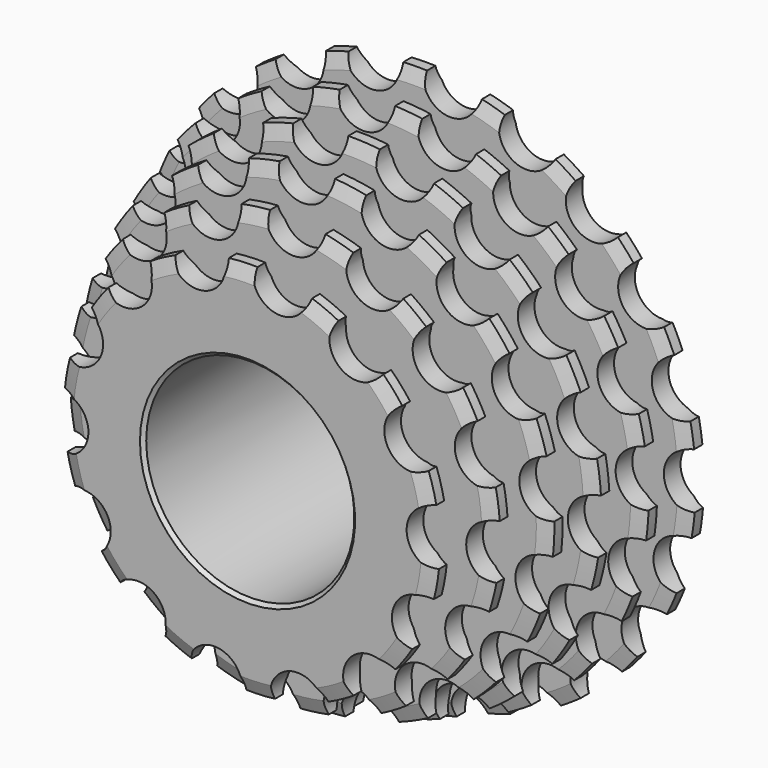
from build123d import *

# Parameters (mm, degrees)
F0_R        = 15
F1_DEPTH    = 3
F2_SIZE2    = 0.75
F2_SIZE     = 2
F2_2_SIZE2  = 0.75
F2_2_SIZE   = 2
F4_SIZE     = 0.5
F5_R        = 17.5
F6_DEPTH    = 3
F7_R        = 38.0209406439
F8_DEPTH    = 3
F9_SIZE2    = 0.75
F9_SIZE     = 2
F9_2_SIZE2  = 0.75
F9_2_SIZE   = 2
F10_R       = 4
F11_DEPTH   = 3
F12_R       = 17.5
F13_DEPTH   = 3
F14_R       = 36.0043728374
F15_DEPTH   = 3
F16_SIZE2   = 2
F16_SIZE    = 0.75
F17_R       = 4
F18_DEPTH   = 3
F19_R       = 17.5
F20_DEPTH   = 3
F21_R       = 34.0193951986
F22_DEPTH   = 3
F23_SIZE2   = 2
F23_SIZE    = 0.75
F24_R       = 4
F25_DEPTH   = 3
F26_R       = 17.5
F27_DEPTH   = 3
F28_R       = 30.9833920726
F29_DEPTH   = 3
F30_SIZE2   = 0.8
F30_SIZE    = 2
F30_2_SIZE2 = 0.8
F30_2_SIZE  = 2
F31_R       = 4
F32_DEPTH   = 3
F33_R       = 17.5
F34_DEPTH   = 3
F35_R       = 27.0849501577
F36_DEPTH   = 3
F37_SIZE2   = 0.8
F37_SIZE    = 2
F37_2_SIZE2 = 0.8
F37_2_SIZE  = 2
F38_R       = 4
F39_DEPTH   = 3
F40_R       = 15
F41_DEPTH   = 30.0010001
F42_SIZE    = 0.5


# Not quite as in the source:
# - two fillets or chamfers of one size are made in one step


with BuildPart() as f1:
    # F0 (on Front) → F1 (new body)
    with BuildSketch(Plane.XZ):
        with BuildLine():
            ThreePointArc((39.8415623905, -3.556670674), (35.9978191055, 0.3962570459), (39.7536154095, 4.4328390311))
            ThreePointArc((39.7536154095, 4.4328390311), (39.5277999491, 6.1280528053), (39.2297290943, 7.8120647197))
            ThreePointArc((39.2297290943, 7.8120647197), (34.4280159865, 10.5219634686), (36.8944395869, 15.4531656165))
            ThreePointArc((36.8944395869, 15.4531656165), (36.2001743283, 17.0160917546), (35.4397364551, 18.5479130899))
            ThreePointArc((35.4397364551, 18.5479130899), (30.0690597635, 19.7952429876), (31.0462956886, 25.2215686272))
            ThreePointArc((31.0462956886, 25.2215686272), (29.9398258742, 26.5255881485), (28.7786271366, 27.7811198502))
            ThreePointArc((28.7786271366, 27.7811198502), (23.2740871461, 27.4648296466), (22.6829655531, 32.9466701461))
            ThreePointArc((22.6829655531, 32.9466701461), (21.2539307867, 33.8861391444), (19.7860446005, 34.763665501))
            ThreePointArc((19.7860446005, 34.763665501), (14.5935864044, 32.9093791473), (12.4819964492, 38.0026283912))
            ThreePointArc((12.4819964492, 38.0026283912), (10.8461686289, 38.5014366755), (9.190514403, 38.9298657204))
            ThreePointArc((9.190514403, 38.9298657204), (4.7308000836, 35.687806469), (1.2698102264, 39.9798396944))
            ThreePointArc((1.2698102264, 39.9798396944), (-0.4402856066, 39.9975767839), (-2.1495766133, 39.9421997439))
            ThreePointArc((-2.1495766133, 39.9421997439), (-2.1334373815, 39.7352791434), (-2.1280528053, 39.5277999491))
            ThreePointArc((-2.1280528053, 39.5277999491), (-5.7211023511, 35.548554879), (-10.0452484692, 38.7181221548))
            ThreePointArc((-10.0452484692, 38.7181221548), (-11.6910705207, 38.2533510961), (-13.3155217164, 37.7186542896))
            ThreePointArc((-13.3155217164, 37.7186542896), (-13.091663124, 36.9740347316), (-13.0160917546, 36.2001743283))
            ThreePointArc((-13.0160917546, 36.2001743283), (-16.0469778506, 32.3193473235), (-20.5465008752, 34.3196926237))
            ThreePointArc((-20.5465008752, 34.3196926237), (-21.9947144307, 33.4100664039), (-23.4027224406, 32.4393677862))
            ThreePointArc((-23.4027224406, 32.4393677862), (-22.751236361, 31.2643139202), (-22.5255881485, 29.9398258742))
            ThreePointArc((-22.5255881485, 29.9398258742), (-25.0140391592, 26.2364193811), (-29.383197975, 27.1408857034))
            ThreePointArc((-29.383197975, 27.1408857034), (-30.5164773851, 25.860096829), (-31.5939737739, 24.5320366291))
            ThreePointArc((-31.5939737739, 24.5320366291), (-30.338699118, 23.1020837184), (-29.8861391444, 21.2539307867))
            ThreePointArc((-29.8861391444, 21.2539307867), (-31.8629258482, 17.8033354818), (-35.8394431235, 17.7632856364))
            ThreePointArc((-35.8394431235, 17.7632856364), (-36.5659768303, 16.2150960049), (-37.2256692487, 14.637265762))
            ThreePointArc((-37.2256692487, 14.637265762), (-35.2531240591, 13.1803633822), (-34.5014366755, 10.8461686289))
            ThreePointArc((-34.5014366755, 10.8461686289), (-36.0077458606, 7.7186286819), (-39.3921897355, 6.9466098095))
            ThreePointArc((-39.3921897355, 6.9466098095), (-39.6531182989, 5.2564445374), (-39.8415623905, 3.556670674))
            ThreePointArc((-39.8415623905, 3.556670674), (-37.1145178551, 2.3324334944), (-35.9975767839, -0.4402856066))
            ThreePointArc((-35.9975767839, -0.4402856066), (-37.0841728042, -3.1811025014), (-39.7536154095, -4.4328390311))
            ThreePointArc((-39.7536154095, -4.4328390311), (-39.5277999491, -6.1280528053), (-39.2297290943, -7.8120647197))
            ThreePointArc((-39.2297290943, -7.8120647197), (-35.7942366206, -8.536271637), (-34.2533510961, -11.6910705207))
            ThreePointArc((-34.2533510961, -11.6910705207), (-34.979542455, -13.9893692353), (-36.8944395869, -15.4531656165))
            ThreePointArc((-36.8944395869, -15.4531656165), (-36.2001743283, -17.0160917546), (-35.4397364551, -18.5479130899))
            ThreePointArc((-35.4397364551, -18.5479130899), (-31.4249568609, -18.5220583719), (-29.4100664039, -21.9947144307))
            ThreePointArc((-29.4100664039, -21.9947144307), (-29.8424984045, -23.803708231), (-31.0462956886, -25.2215686272))
            ThreePointArc((-31.0462956886, -25.2215686272), (-29.9398258742, -26.5255881485), (-28.7786271366, -27.7811198502))
            ThreePointArc((-28.7786271366, -27.7811198502), (-24.3894033243, -26.7966574143), (-21.860096829, -30.5164773851))
            ThreePointArc((-21.860096829, -30.5164773851), (-22.0713948676, -31.799340374), (-22.6829655531, -32.9466701461))
            ThreePointArc((-22.6829655531, -32.9466701461), (-21.2539307867, -33.8861391444), (-19.7860446005, -34.763665501))
            ThreePointArc((-19.7860446005, -34.763665501), (-15.288757617, -32.674717755), (-12.2150960049, -36.5659768303))
            ThreePointArc((-12.2150960049, -36.5659768303), (-12.2823871279, -37.2965936168), (-12.4819964492, -38.0026283912))
            ThreePointArc((-12.4819964492, -38.0026283912), (-10.8461686289, -38.5014366755), (-9.190514403, -38.9298657204))
            ThreePointArc((-9.190514403, -38.9298657204), (-4.8933188446, -35.6696349324), (-1.2564445374, -39.6531182989))
            ThreePointArc((-1.2564445374, -39.6531182989), (-1.2597873564, -39.8166156321), (-1.2698102264, -39.9798396944))
            ThreePointArc((-1.2698102264, -39.9798396944), (0.4402856066, -39.9975767839), (2.1495766133, -39.9421997439))
            ThreePointArc((2.1495766133, -39.9421997439), (5.5152475248, -35.5750199542), (10.0452484692, -38.7181221548))
            ThreePointArc((10.0452484692, -38.7181221548), (11.6910705207, -38.2533510961), (13.3155217164, -37.7186542896))
            ThreePointArc((13.3155217164, -37.7186542896), (15.3144825791, -32.5801568955), (20.5465008752, -34.3196926237))
            ThreePointArc((20.5465008752, -34.3196926237), (21.9947144307, -33.4100664039), (23.4027224406, -32.4393677862))
            ThreePointArc((23.4027224406, -32.4393677862), (23.8730293337, -26.9458432867), (29.383197975, -27.1408857034))
            ThreePointArc((29.383197975, -27.1408857034), (30.5164773851, -25.860096829), (31.5939737739, -24.5320366291))
            ThreePointArc((31.5939737739, -24.5320366291), (30.49752523, -19.128537708), (35.8394431235, -17.7632856364))
            ThreePointArc((35.8394431235, -17.7632856364), (36.5659768303, -16.2150960049), (37.2256692487, -14.637265762))
            ThreePointArc((37.2256692487, -14.637265762), (34.6512930079, -9.761551766), (39.3921897355, -6.9466098095))
            ThreePointArc((39.3921897355, -6.9466098095), (39.6531182989, -5.2564445374), (39.8415623905, -3.556670674))
        make_face()
        Circle(F0_R, mode=Mode.SUBTRACT)
    extrude(amount=F1_DEPTH)

    # F2
    f2_edges = [f1.edges().sort_by_distance(p)[0] for p in [
        (-10.846169, 0, -38.501437),
        (-21.253931, 0, -33.886139),
        (-29.939826, 0, -26.525588),
        (-36.200174, 0, -17.016092),
        (-39.5278, 0, -6.128053),
        (-39.653118, 0, 5.256445),
        (-36.565977, 0, 16.215096),
        (-30.516477, 0, 25.860097),
        (-21.994714, 0, 33.410066),
        (-11.691071, 0, 38.253351),
        (-0.440286, 0, 39.997577),
        (10.846169, 0, 38.501437),
        (21.253931, 0, 33.886139),
        (29.939826, 0, 26.525588),
        (36.200174, 0, 17.016092),
        (39.5278, 0, 6.128053),
        (39.653118, 0, -5.256445),
        (36.565977, 0, -16.215096),
        (30.516477, 0, -25.860097),
        (21.994714, 0, -33.410066),
        (11.691071, 0, -38.253351),
        (0.440286, 0, -39.997577),
    ]]
    f2_side = f1.faces().sort_by_distance((-10.54, 0, -37.414606))[0]
    chamfer(f2_edges, length=F2_SIZE, length2=F2_SIZE2, reference=f2_side)

    # F2#2
    f2_2_edges = [f1.edges().sort_by_distance(p)[0] for p in [
        (-10.846169, -3, -38.501437),
        (0.440286, -3, -39.997577),
        (11.691071, -3, -38.253351),
        (21.994714, -3, -33.410066),
        (30.516477, -3, -25.860097),
        (36.565977, -3, -16.215096),
        (39.653118, -3, -5.256445),
        (39.5278, -3, 6.128053),
        (36.200174, -3, 17.016092),
        (29.939826, -3, 26.525588),
        (21.253931, -3, 33.886139),
        (10.846169, -3, 38.501437),
        (-0.440286, -3, 39.997577),
        (-11.691071, -3, 38.253351),
        (-21.994714, -3, 33.410066),
        (-30.516477, -3, 25.860097),
        (-36.565977, -3, 16.215096),
        (-39.653118, -3, 5.256445),
        (-39.5278, -3, -6.128053),
        (-36.200174, -3, -17.016092),
        (-29.939826, -3, -26.525588),
        (-21.253931, -3, -33.886139),
    ]]
    f2_2_side = f1.faces().sort_by_distance((-10.54, -3, -37.414606))[0]
    chamfer(f2_2_edges, length=F2_2_SIZE, length2=F2_2_SIZE2, reference=f2_2_side)

    # F4
    f4_edges = [f1.edges().sort_by_distance(p)[0] for p in [
        (-15, -3, 0),
        (-15, 0, 0),
    ]]
    chamfer(f4_edges, length=F4_SIZE)

    # F5 (on face) → F6 (join)
    with BuildSketch(Plane.XZ.offset(3)):
        Circle(F5_R)
    extrude(amount=F6_DEPTH)

    # F7 (on face) → F8 (join)
    with BuildSketch(Plane.XZ.offset(6)):
        Circle(F7_R)
    extrude(amount=F8_DEPTH)

    # F9
    f9_edges = [f1.edges().sort_by_distance(p)[0] for p in [
        (-38.020941, -9, 0),
    ]]
    f9_side = f1.faces().sort_by_distance((0, -9, 0))[0]
    chamfer(f9_edges, length=F9_SIZE, length2=F9_SIZE2, reference=f9_side)

    # F9#2
    f9_2_edges = [f1.edges().sort_by_distance(p)[0] for p in [
        (-38.020941, -6, 0),
    ]]
    f9_2_side = f1.faces().sort_by_distance((-36.945546, -6, 0))[0]
    chamfer(f9_2_edges, length=F9_2_SIZE, length2=F9_2_SIZE2, reference=f9_2_side)

    # F10 (on face) → F11 (cut)
    with BuildSketch(Plane.XZ.offset(9)):
        with Locations((-32.1056060493, 20.1982129365)):
            Circle(F10_R)
        with Locations((-36.7758368962, 9.2884641469)):
            Circle(F10_R)
        with Locations((-37.8461925953, -2.53050423)):
            Circle(F10_R)
        with Locations((-35.2118992733, -14.1017692218)):
            Circle(F10_R)
        with Locations((-29.1308199147, -24.2926547894)):
            Circle(F10_R)
        with Locations((-20.1982129365, -32.1056060493)):
            Circle(F10_R)
        with Locations((-9.2884641469, -36.7758368962)):
            Circle(F10_R)
        with Locations((2.53050423, -37.8461925953)):
            Circle(F10_R)
        with Locations((14.1017692218, -35.2118992733)):
            Circle(F10_R)
        with Locations((24.2926547894, -29.1308199147)):
            Circle(F10_R)
        with Locations((32.1056060493, -20.1982129365)):
            Circle(F10_R)
        with Locations((36.7758368962, -9.2884641469)):
            Circle(F10_R)
        with Locations((37.8461925953, 2.53050423)):
            Circle(F10_R)
        with Locations((35.2118992733, 14.1017692218)):
            Circle(F10_R)
        with Locations((29.1308199147, 24.2926547894)):
            Circle(F10_R)
        with Locations((20.1982129365, 32.1056060493)):
            Circle(F10_R)
        with Locations((9.2884641469, 36.7758368962)):
            Circle(F10_R)
        with Locations((-2.53050423, 37.8461925953)):
            Circle(F10_R)
        with Locations((-14.1017692218, 35.2118992733)):
            Circle(F10_R)
        with Locations((-24.2926547894, 29.1308199147)):
            Circle(F10_R)
    extrude(amount=-F11_DEPTH, mode=Mode.SUBTRACT)

    # F12 (on face) → F13 (join)
    with BuildSketch(Plane.XZ.offset(9)):
        Circle(F12_R)
    extrude(amount=F13_DEPTH)

    # F14 (on face) → F15 (join)
    with BuildSketch(Plane.XZ.offset(12)):
        Circle(F14_R)
    extrude(amount=F15_DEPTH)

    # F16
    f16_edges = [f1.edges().sort_by_distance(p)[0] for p in [
        (-36.004373, -15, 0),
        (-36.004373, -12, 0),
    ]]
    f16_side = f1.faces().sort_by_distance((-36.004373, -13.5, 0))[0]
    chamfer(f16_edges, length=F16_SIZE, length2=F16_SIZE2, reference=f16_side)

    # F17 (on face) → F18 (cut)
    with BuildSketch(Plane.XZ.offset(15)):
        with Locations((-26.2372046709, 24.3606828153)):
            Circle(F17_R)
        with Locations((-32.9867518473, 13.9179013768)):
            Circle(F17_R)
        with Locations((-35.7576099183, 1.796415626)):
            Circle(F17_R)
        with Locations((-34.215572507, -10.5417443616)):
            Circle(F17_R)
        with Locations((-28.5466320834, -21.6084143997)):
            Circle(F17_R)
        with Locations((-19.434546527, -30.0687907549)):
            Circle(F17_R)
        with Locations((-7.9783678361, -34.902427177)):
            Circle(F17_R)
        with Locations((4.4401197639, -35.5263157765)):
            Circle(F17_R)
        with Locations((16.3230633913, -31.8652063809)):
            Circle(F17_R)
        with Locations((26.2372046709, -24.3606828153)):
            Circle(F17_R)
        with Locations((32.9867518473, -13.9179013768)):
            Circle(F17_R)
        with Locations((35.7576099183, -1.796415626)):
            Circle(F17_R)
        with Locations((34.215572507, 10.5417443616)):
            Circle(F17_R)
        with Locations((28.5466320834, 21.6084143997)):
            Circle(F17_R)
        with Locations((19.434546527, 30.0687907549)):
            Circle(F17_R)
        with Locations((7.9783678361, 34.902427177)):
            Circle(F17_R)
        with Locations((-4.4401197639, 35.5263157765)):
            Circle(F17_R)
        with Locations((-16.3230633913, 31.8652063809)):
            Circle(F17_R)
    extrude(amount=-F18_DEPTH, mode=Mode.SUBTRACT)

    # F19 (on face) → F20 (join)
    with BuildSketch(Plane.XZ.offset(15)):
        Circle(F19_R)
    extrude(amount=F20_DEPTH)

    # F21 (on face) → F22 (join)
    with BuildSketch(Plane.XZ.offset(18)):
        Circle(F21_R)
    extrude(amount=F22_DEPTH)

    # F23
    f23_edges = [f1.edges().sort_by_distance(p)[0] for p in [
        (-34.019395, -21, 0),
        (-34.019395, -18, 0),
    ]]
    f23_side = f1.faces().sort_by_distance((-34.019395, -19.5, 0))[0]
    chamfer(f23_edges, length=F23_SIZE, length2=F23_SIZE2, reference=f23_side)

    # F24 (on face) → F25 (cut)
    with BuildSketch(Plane.XZ.offset(21)):
        with Locations((-23.9853784442, 23.951260373)):
            Circle(F24_R)
        with Locations((-31.0178925154, 13.6693670837)):
            Circle(F24_R)
        with Locations((-33.8612683263, 1.5413500253)):
            Circle(F24_R)
        with Locations((-32.131492218, -10.7948348951)):
            Circle(F24_R)
        with Locations((-26.0621800389, -21.6731175466)):
            Circle(F24_R)
        with Locations((-16.47302603, -29.6243255785)):
            Circle(F24_R)
        with Locations((-4.6590985756, -33.574604287)):
            Circle(F24_R)
        with Locations((7.7840659584, -32.9904466433)):
            Circle(F24_R)
        with Locations((19.1759492517, -27.9507463739)):
            Circle(F24_R)
        with Locations((27.978014341, -19.1361429264)):
            Circle(F24_R)
        with Locations((33.001493562, -7.7370973396)):
            Circle(F24_R)
        with Locations((33.5679382099, 4.7068861156)):
            Circle(F24_R)
        with Locations((29.6008467961, 16.5151785192)):
            Circle(F24_R)
        with Locations((21.6359969986, 26.0930045499)):
            Circle(F24_R)
        with Locations((10.7490859172, 32.1468257299)):
            Circle(F24_R)
        with Locations((-1.58954878, 33.8590399634)):
            Circle(F24_R)
        with Locations((-13.7135061065, 30.9984032304)):
            Circle(F24_R)
    extrude(amount=-F25_DEPTH, mode=Mode.SUBTRACT)

    # F26 (on face) → F27 (join)
    with BuildSketch(Plane.XZ.offset(21)):
        Circle(F26_R)
    extrude(amount=F27_DEPTH)

    # F28 (on face) → F29 (join)
    with BuildSketch(Plane.XZ.offset(24)):
        Circle(F28_R)
    extrude(amount=F29_DEPTH)

    # F30
    f30_edges = [f1.edges().sort_by_distance(p)[0] for p in [
        (-30.983392, -27, 0),
    ]]
    f30_side = f1.faces().sort_by_distance((0, -27, 0))[0]
    chamfer(f30_edges, length=F30_SIZE, length2=F30_SIZE2, reference=f30_side)

    # F30#2
    f30_2_edges = [f1.edges().sort_by_distance(p)[0] for p in [
        (-30.983392, -24, 0),
    ]]
    f30_2_side = f1.faces().sort_by_distance((-30.107049, -24, 0))[0]
    chamfer(f30_2_edges, length=F30_2_SIZE, length2=F30_2_SIZE2, reference=f30_2_side)

    # F31 (on face) → F32 (cut)
    with BuildSketch(Plane.XZ.offset(27)):
        with Locations((-20.4370431602, 22.9959394783)):
            Circle(F31_R)
        with Locations((-27.6815309308, 13.4245599909)):
            Circle(F31_R)
        with Locations((-30.7117565508, 1.8094129389)):
            Circle(F31_R)
        with Locations((-29.0663956388, -10.0812008308)):
            Circle(F31_R)
        with Locations((-22.9959394783, -20.4370431602)):
            Circle(F31_R)
        with Locations((-13.4245599909, -27.6815309308)):
            Circle(F31_R)
        with Locations((-1.8094129389, -30.7117565508)):
            Circle(F31_R)
        with Locations((10.0812008308, -29.0663956388)):
            Circle(F31_R)
        with Locations((20.4370431602, -22.9959394783)):
            Circle(F31_R)
        with Locations((27.6815309308, -13.4245599909)):
            Circle(F31_R)
        with Locations((30.7117565508, -1.8094129389)):
            Circle(F31_R)
        with Locations((29.0663956388, 10.0812008308)):
            Circle(F31_R)
        with Locations((22.9959394783, 20.4370431602)):
            Circle(F31_R)
        with Locations((13.4245599909, 27.6815309308)):
            Circle(F31_R)
        with Locations((1.8094129389, 30.7117565508)):
            Circle(F31_R)
        with Locations((-10.0812008308, 29.0663956388)):
            Circle(F31_R)
    extrude(amount=-F32_DEPTH, mode=Mode.SUBTRACT)

    # F33 (on face) → F34 (join)
    with BuildSketch(Plane.XZ.offset(27)):
        Circle(F33_R)
    extrude(amount=F34_DEPTH)

    # F35 (on face) → F36 (join)
    with BuildSketch(Plane.XZ.offset(30)):
        Circle(F35_R)
    extrude(amount=F36_DEPTH)

    # F37
    f37_edges = [f1.edges().sort_by_distance(p)[0] for p in [
        (-27.08495, -33, 0),
    ]]
    f37_side = f1.faces().sort_by_distance((0, -33, 0))[0]
    chamfer(f37_edges, length=F37_SIZE, length2=F37_SIZE2, reference=f37_side)

    # F37#2
    f37_2_edges = [f1.edges().sort_by_distance(p)[0] for p in [
        (-27.08495, -30, 0),
    ]]
    f37_2_side = f1.faces().sort_by_distance((-26.318872, -30, 0))[0]
    chamfer(f37_2_edges, length=F37_2_SIZE, length2=F37_2_SIZE2, reference=f37_2_side)

    # F38 (on face) → F39 (cut)
    with BuildSketch(Plane.XZ.offset(33)):
        with Locations((-17.7757926285, 20.2664509416)):
            Circle(F38_R)
        with Locations((-24.8087192738, 10.5468139898)):
            Circle(F38_R)
        with Locations((-26.9279748078, -1.2617488209)):
            Circle(F38_R)
        with Locations((-23.7138146813, -12.8204068032)):
            Circle(F38_R)
        with Locations((-15.8028427263, -21.8398259862)):
            Circle(F38_R)
        with Locations((-4.7619239602, -26.5335997847)):
            Circle(F38_R)
        with Locations((7.2221522474, -25.9720687327)):
            Circle(F38_R)
        with Locations((17.7757926285, -20.2664509416)):
            Circle(F38_R)
        with Locations((24.8087192738, -10.5468139898)):
            Circle(F38_R)
        with Locations((26.9279748078, 1.2617488209)):
            Circle(F38_R)
        with Locations((23.7138146813, 12.8204068032)):
            Circle(F38_R)
        with Locations((15.8028427263, 21.8398259862)):
            Circle(F38_R)
        with Locations((4.7619239602, 26.5335997847)):
            Circle(F38_R)
        with Locations((-7.2221522474, 25.9720687327)):
            Circle(F38_R)
    extrude(amount=-F39_DEPTH, mode=Mode.SUBTRACT)

    # F40 (on face) → F41 (cut, through all)
    with BuildSketch(Plane(origin=(0, -3, 0), x_dir=(-1, 0, 0), z_dir=(0, 1, 0))):
        Circle(F40_R)
    extrude(amount=-F41_DEPTH, mode=Mode.SUBTRACT)

    # F42
    f42_edges = [f1.edges().sort_by_distance(p)[0] for p in [
        (15, -33, 0),
    ]]
    chamfer(f42_edges, length=F42_SIZE)


solid = f1.part
